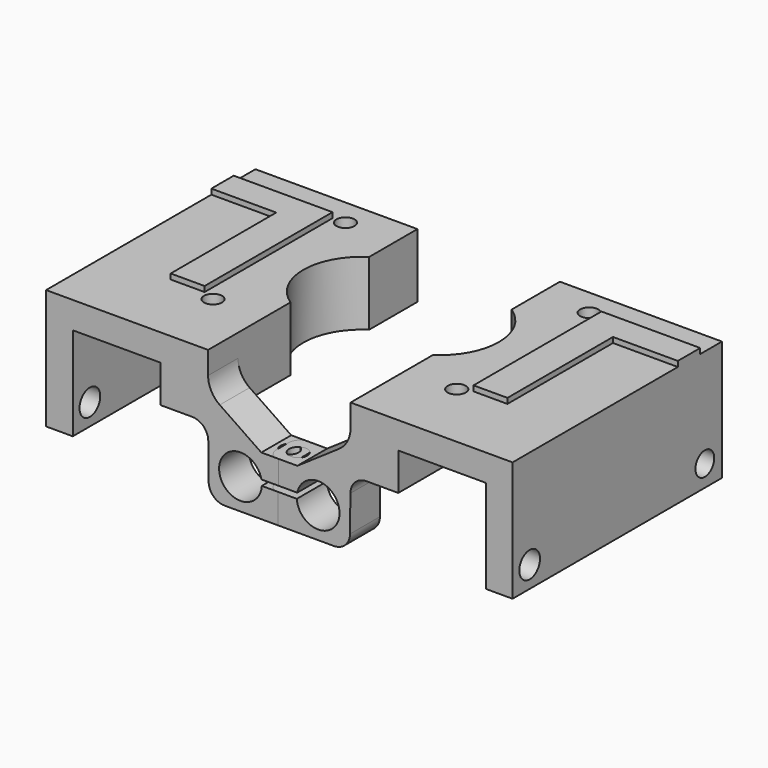
from build123d import *

# Parameters (mm, degrees)
F1_DEPTH      = 7
F2_DEPTH      = 42
F3_R          = 1.7
F3_R_2        = 11
F4_DEPTH      = 12.001
F5_R          = 4
F6_DEPTH      = 10
F7_DEPTH      = 12.001
F8_R          = 1.4
F9_DEPTH      = 10.9920075553
F8_R_2        = 1.7
F10_DEPTH     = 4.4348209087
F11_R         = 5
F12_R         = 3
F13_R         = 3
F14_R         = 2
F15_R         = 2.2
F15_R_2       = 2.4255023423
F16_DEPTH     = 6
F17_TEXT_SIZE = 41.9437823343
F18_DEPTH     = 1


# Not quite as in the source:
# - a feature names something its author has since deleted; it is built from what else it names
# - Text() gives the source's letters only with a copy of the font that has no kerning and outlines rounded to 1/6400 em; it was checked with that copy


with BuildPart() as f1:
    # F0 (on Front) → F1 (new body)
    with BuildSketch(Plane.XZ):
        Polygon((-18.6721007523, 29.8099789735), (-18.6721007523, 7.3259699669), (-13.6721007523, 7.3259699669), (-13.6721007523, 24.8099789735), (2.7278992477, 24.8099789735), (2.7278992477, 17.8099789735), (11.6637966118, 17.8099789735), (11.6637966118, 22.9406704692), (11.6637966118, 29.8099789735), align=None)
        Polygon((21.6301751077, 16.1394868046), (11.6637966118, 22.9406704692), (11.6637966118, 17.8099789735), (11.7940201178, 5.1484792493), (27.2186601057, 5.1484792493), (27.2186601057, 10.6682249423), (19.8860510706, 10.6682249423), (19.8860510706, 11.7046658959), (27.1896428882, 11.7046658959), (27.1896428882, 16.1394868046), align=None)
    extrude(amount=F1_DEPTH)

    # F0 (on Front) → F2 (join)
    with BuildSketch(Plane.XZ):
        Polygon((-18.6721007523, 29.8099789735), (-18.6721007523, 7.3259699669), (-13.6721007523, 7.3259699669), (-13.6721007523, 24.8099789735), (2.7278992477, 24.8099789735), (2.7278992477, 17.8099789735), (11.6637966118, 17.8099789735), (11.6637966118, 22.9406704692), (11.6637966118, 29.8099789735), align=None)
    extrude(amount=-F2_DEPTH)

    # F3 (on face) → F4 (cut, through all)
    with BuildSketch(Plane(origin=(0, 0, 17.8099789735), x_dir=(1, 0, 0), z_dir=(0, 0, -1))):
        with Locations((2.1850741468, -6)):
            Circle(F3_R)
        with Locations((2.1850741468, -37)):
            Circle(F3_R)
        with Locations((17.6850741468, -21.5)):
            Circle(F3_R_2)
    extrude(amount=-F4_DEPTH, mode=Mode.SUBTRACT)

    # F5 (on face) → F6 (cut)
    with BuildSketch(Plane.XZ.offset(7)):
        with Locations((17.7278992477, 10.8989789735)):
            Circle(F5_R)
    extrude(amount=-F6_DEPTH, mode=Mode.SUBTRACT)

    # F3 (on face) → F7 (cut, through all)
    with BuildSketch(Plane(origin=(0, 0, 17.8099789735), x_dir=(1, 0, 0), z_dir=(0, 0, -1))):
        with Locations((2.1850741468, -6)):
            Circle(F3_R)
        with Locations((2.1850741468, -37)):
            Circle(F3_R)
        with Locations((17.6850741468, -21.5)):
            Circle(F3_R_2)
    extrude(amount=-F7_DEPTH, mode=Mode.SUBTRACT)

    # F8 (on face) → F9 (cut, through all)
    with BuildSketch(Plane.XY.offset(16.1394868046)):
        with Locations((24.1896428882, -3.5767070949)):
            Circle(F8_R)
    extrude(amount=-F9_DEPTH, mode=Mode.SUBTRACT)

    # F8 (on face) → F10 (cut, through all)
    with BuildSketch(Plane.XY.offset(16.1394868046)):
        with Locations((24.1896428882, -3.5767070949)):
            Circle(F8_R_2)
        with Locations((24.1896428882, -3.5767070949)):
            Circle(F8_R, mode=Mode.SUBTRACT)
    extrude(amount=-F10_DEPTH, mode=Mode.SUBTRACT)

    # F11
    f11_edges = [f1.edges().sort_by_distance(p)[0] for p in [
        (11.663797, -3.5, 22.94067),
    ]]
    fillet(f11_edges, radius=F11_R)

    # F12
    f12_edges = [f1.edges().sort_by_distance(p)[0] for p in [
        (11.663797, -3.5, 17.809979),
    ]]
    fillet(f12_edges, radius=F12_R)

    # F13
    f13_edges = [f1.edges().sort_by_distance(p)[0] for p in [
        (11.79402, -3.5, 5.148479),
    ]]
    fillet(f13_edges, radius=F13_R)

    # F14
    f14_edges = [f1.edges().sort_by_distance(p)[0] for p in [
        (27.189643, -7, 13.922076),
        (27.21866, -7, 7.908352),
        (27.189643, 0, 13.922076),
        (27.21866, 0, 7.908352),
    ]]
    fillet(f14_edges, radius=F14_R)

    # F15 (on face) → F16 (cut)
    with BuildSketch(Plane(origin=(-18.6721007523, 0, 0), x_dir=(0, -1, 0), z_dir=(-1, 0, 0))):
        with Locations((-38, 11.3259699669)):
            Circle(F15_R)
        with Locations((3, 11.3259699669)):
            Circle(F15_R_2)
    extrude(amount=-F16_DEPTH, mode=Mode.SUBTRACT)

    # F17 (on face) → F18 (join)
    with BuildSketch(Plane.XY.offset(29.8099789735)):
        with Locations(Location((3.5908724648, 36.9253193088), (0, 0, 180))):
            Text('L', F17_TEXT_SIZE, font='Open Sans', font_style=FontStyle.BOLD, text_align=(TextAlign.LEFT, TextAlign.BOTTOM))
    extrude(amount=F18_DEPTH)


with BuildPart() as f19_1:
    # F19: instance of F1
    add(f1.part.mirror(Plane.YZ))


with BuildPart() as f19_1_1:
    # F20: moved
    add(f19_1.part.moved(Location((50, 0, 0))))


solid = Compound([f1.part, f19_1_1.part])
